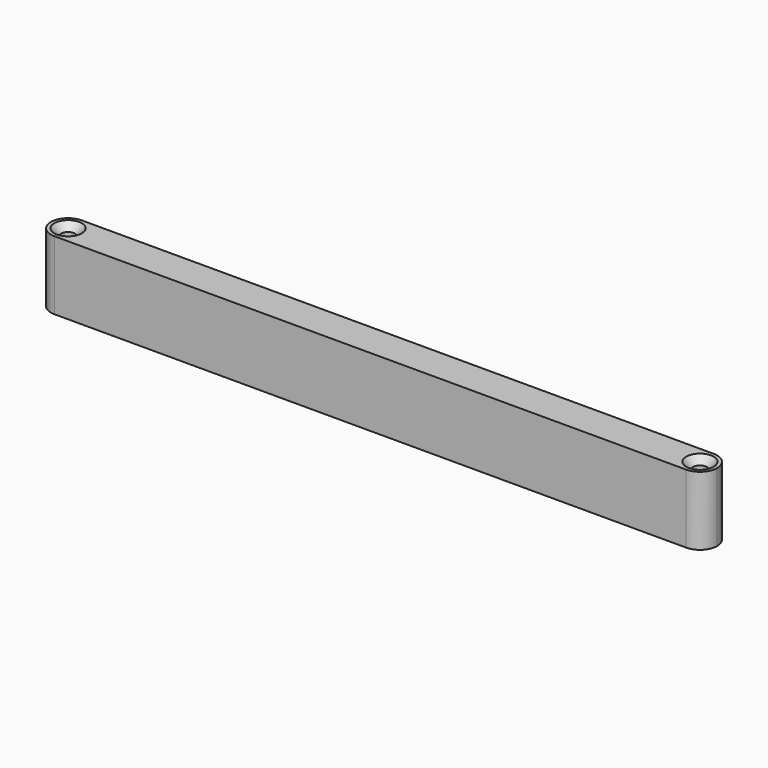
from build123d import *

# Parameters (mm, degrees)
F0_W     = 97
F0_H     = 5
F0_R     = 1
F1_DEPTH = 10
F2_R     = 2.49999
F3_SIZE  = 1


# Not quite as in the source:
# - a fillet or chamfer is up to 0.001 mm smaller than in the source, because OpenCascade refuses the exact size


with BuildPart() as f1:
    # F0 (on Top) → F1 (new body)
    with BuildSketch(Plane.XY):
        Rectangle(F0_W, F0_H)
        with Locations((-46, 0)):
            Circle(F0_R, mode=Mode.SUBTRACT)
        with Locations((46, 0)):
            Circle(F0_R, mode=Mode.SUBTRACT)
    extrude(amount=F1_DEPTH)

    # F2 (radius 2.5 in the source; OpenCascade refuses exactly that, so slightly less here)
    f2_edges = [f1.edges().sort_by_distance(p)[0] for p in [
        (48.5, 2.5, 5),
        (48.5, -2.5, 5),
        (-48.5, 2.5, 5),
        (-48.5, -2.5, 5),
    ]]
    fillet(f2_edges, radius=F2_R)

    # F3
    f3_edges = [f1.edges().sort_by_distance(p)[0] for p in [
        (-47, 0, 10),
        (45, 0, 10),
        (45, 0, 0),
        (-47, 0, 0),
    ]]
    chamfer(f3_edges, length=F3_SIZE)


solid = f1.part
